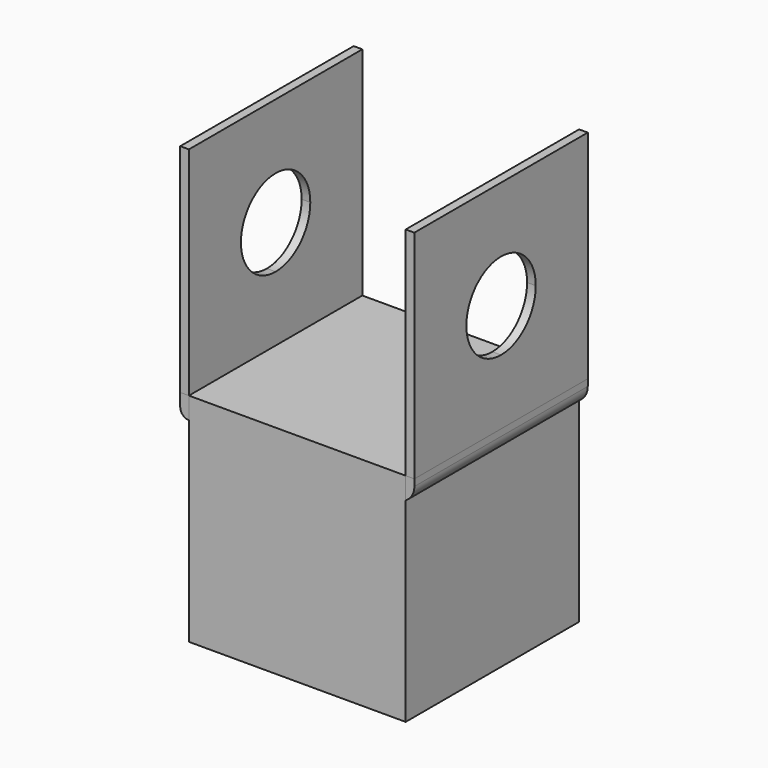
from build123d import *

# Parameters (mm, degrees)
F0_W         = 63.5
F0_H         = 63.5
F1_DEPTH     = 127
F2_W         = 63.5
F2_H         = 63.5
F3_DEPTH     = 2.54
F5_DEPTH     = 2.54
F7_DEPTH     = 2.54
F8_W         = 2.54
F8_H         = 63.5
F8_W_2       = 63.5
F9_DEPTH     = 2.54
F10_W        = 63.5
F10_H        = 63.5
F11_DEPTH    = 63.501
F12_DEPTH    = 6.35
F13_R        = 2.53999
F14_T1_DEPTH = 85.4970452561
F16_DEPTH    = 127
F18_DEPTH    = 25.4


# Not quite as in the source:
# - a fillet or chamfer that OpenCascade refuses, or shapes differently, is made with other operations: its cross-section is extruded or revolved along the edge and cut away or added
# - a fillet or chamfer is up to 0.001 mm smaller than in the source, because OpenCascade refuses the exact size


with BuildPart() as f1:
    # F0 (on Top) → F1 (new body)
    with BuildSketch(Plane.XY):
        with Locations((-46.4062093869, 38.1102421433)):
            Rectangle(F0_W, F0_H)
    extrude(amount=F1_DEPTH)

    # F2 (on face) → F3 (join)
    with BuildSketch(Plane(origin=(0, 69.8602421433, 0), x_dir=(-1, 0, 0), z_dir=(0, 1, 0))):
        with Locations((46.4062093869, 95.25)):
            Rectangle(F2_W, F2_H)
    extrude(amount=F3_DEPTH)


with BuildPart() as f5:
    # F4 (on face) → F5 (new body)
    with BuildSketch(Plane(origin=(-78.1562093869, 0, 0), x_dir=(0, -1, 0), z_dir=(-1, 0, 0))):
        Polygon((-6.3602421433, 127), (-72.4002421433, 127), (-72.4002421433, 63.5), (-69.8602421433, 63.5), (-6.3602421433, 63.5), align=None)
    extrude(amount=F5_DEPTH)


with BuildPart() as f7:
    # F6 (on face) → F7 (new body)
    with BuildSketch(Plane.YZ.offset(-14.6562093869)):
        Polygon((72.4002421433, 127), (6.3602421433, 127), (6.3602421433, 63.5), (69.8602421433, 63.5), (72.4002421433, 63.5), align=None)
    extrude(amount=F7_DEPTH)


with BuildPart() as f9_tool:
    # F8 (on face) → F9 (new body)
    with BuildSketch(Plane(origin=(0, 72.4002421433, 0), x_dir=(-1, 0, 0), z_dir=(0, 1, 0))):
        with Locations((13.3862093869, 95.25)):
            Rectangle(F8_W, F8_H)
        with Locations((46.4062093869, 95.25)):
            Rectangle(F8_W_2, F8_H)
        with Locations((79.4262093869, 95.25)):
            Rectangle(F8_W, F8_H)
    extrude(amount=-F9_DEPTH)


with BuildPart() as f1_1:
    add(f1.part)

    # F9: cut by f9_tool
    add(f9_tool.part, mode=Mode.SUBTRACT)

    # F10 (on face) → F11 (cut, through all)
    with BuildSketch(Plane.XZ.offset(-6.3602421433)):
        with Locations((-46.4062093869, 95.25)):
            Rectangle(F10_W, F10_H)
    extrude(amount=-F11_DEPTH, mode=Mode.SUBTRACT)

    # F17 (on face) → F18 (cut)
    with BuildSketch(Plane(origin=(-80.6962093869, 0, 0), x_dir=(0, -1, 0), z_dir=(-1, 0, 0))):
        with BuildLine():
            Line((-38.1102421433, 95.25), (-38.1102421433, 107.95))
            ThreePointArc((-38.1102421433, 107.95), (-47.0904982643, 104.2302561211), (-50.8102421433, 95.25))
            Line((-50.8102421433, 95.25), (-38.1102421433, 95.25))
        make_face()
        with BuildLine():
            Line((-38.1102421433, 95.25), (-50.8102421433, 95.25))
            ThreePointArc((-50.8102421433, 95.25), (-47.0904982643, 86.2697438789), (-38.1102421433, 82.55))
            Line((-38.1102421433, 82.55), (-38.1102421433, 95.25))
        make_face()
        with BuildLine():
            ThreePointArc((-25.4102421433, 95.25), (-29.1299860222, 104.2302561211), (-38.1102421433, 107.95))
            Line((-38.1102421433, 107.95), (-38.1102421433, 95.25))
            Line((-38.1102421433, 95.25), (-38.1102421433, 82.55))
            ThreePointArc((-38.1102421433, 82.55), (-29.1299860222, 86.2697438789), (-25.4102421433, 95.25))
        make_face()
    extrude(amount=-F18_DEPTH, mode=Mode.SUBTRACT)


with BuildPart() as f5_1:
    add(f5.part)

    # F9: cut by f9_tool
    add(f9_tool.part, mode=Mode.SUBTRACT)


with BuildPart() as f7_1:
    add(f7.part)

    # F9: cut by f9_tool
    add(f9_tool.part, mode=Mode.SUBTRACT)


with BuildPart() as f12:
    # F12 (new): a face of the model
    f12_faces = [f5_1.part.faces().sort_by_distance(p)[0] for p in [
        (-79.4262093869, 38.1102421433, 63.5),
    ]]
    extrude(f12_faces, amount=F12_DEPTH)

    # F13 (radius 2.54 in the source; OpenCascade refuses exactly that, so slightly less here)
    f13_edges = [f12.edges().sort_by_distance(p)[0] for p in [
        (-80.696209, 38.110242, 57.15),
    ]]
    fillet(f13_edges, radius=F13_R)


with BuildPart() as f12b:
    # F12#2 (new): a face of the model
    f12_2_faces = [f7_1.part.faces().sort_by_distance(p)[0] for p in [
        (-13.3862093869, 38.1102421433, 63.5),
    ]]
    extrude(f12_2_faces, amount=F12_DEPTH)

    # F14: fillet of radius 5.08 on 1 edges, made by hand

    # F14_s2 → F14_t1 (cut)
    with BuildSketch(Plane.XZ.offset(-80.8587647713)):
        with BuildLine():
            ThreePointArc((-12.1162093869, 61.5494090512), (-12.7968003357, 59.0094090512), (-14.6562093869, 57.15))
            Line((-14.6562093869, 57.15), (-12.1162093869, 57.15))
            Line((-12.1162093869, 57.15), (-12.1162093869, 61.5494090512))
        make_face()
    extrude(amount=F14_T1_DEPTH, mode=Mode.SUBTRACT)


with BuildPart() as f16_tool:
    # F15 (on face) → F16 (new body)
    with BuildSketch(Plane.YZ.offset(-12.1162093869)):
        with BuildLine():
            Line((38.1102421433, 95.25), (38.1102421433, 107.95))
            ThreePointArc((38.1102421433, 107.95), (25.4102421433, 95.25), (38.1102421433, 82.55))
            Line((38.1102421433, 82.55), (38.1102421433, 95.25))
        make_face()
        with BuildLine():
            ThreePointArc((50.8102421433, 95.25), (47.0904982643, 104.2302561211), (38.1102421433, 107.95))
            Line((38.1102421433, 107.95), (38.1102421433, 95.25))
            Line((38.1102421433, 95.25), (38.1102421433, 82.55))
            ThreePointArc((38.1102421433, 82.55), (47.0904982643, 86.2697438789), (50.8102421433, 95.25))
        make_face()
    extrude(amount=-F16_DEPTH)


with BuildPart() as f5_2:
    add(f5_1.part)

    # F16: cut by f16_tool
    add(f16_tool.part, mode=Mode.SUBTRACT)


with BuildPart() as f7_2:
    add(f7_1.part)

    # F16: cut by f16_tool
    add(f16_tool.part, mode=Mode.SUBTRACT)


solid = Compound([f1_1.part, f12.part, f12b.part, f5_2.part, f7_2.part])
